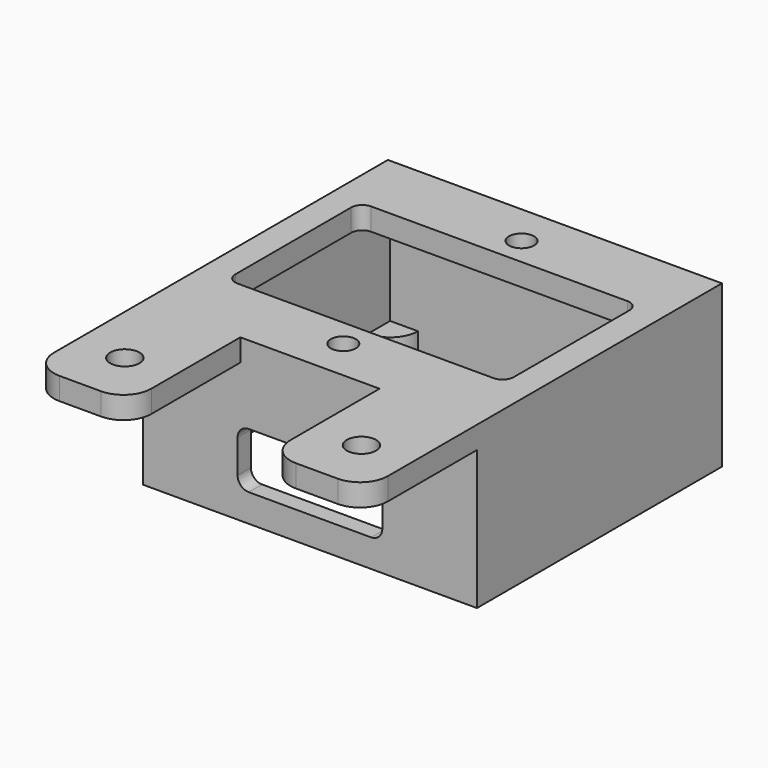
from build123d import *

# Parameters (mm, degrees)
F0_R     = 2.25
F0_R_2   = 2.625
F1_DEPTH = 4
F2_W     = 60
F2_H     = 55
F2_W_2   = 56
F2_H_2   = 50
F3_DEPTH = 25
F5_DEPTH = 25
F6_W     = 5
F6_H     = 5
F7_DEPTH = 5
F8_W     = 56
F8_H     = 50
F9_DEPTH = 2
F10_R    = 4.99999


# Not quite as in the source:
# - a fillet or chamfer is up to 0.001 mm smaller than in the source, because OpenCascade refuses the exact size


with BuildPart() as f1:
    # F0 (on Top) → F1 (new body)
    with BuildSketch(Plane.XY):
        Polygon((30, 27.5), (-30, 27.5), (-30, -27.5), (-12.5000044162, -27.5), (12.5, -27.5), (30, -27.5), align=None)
        with Locations((0, -20)):
            Circle(F0_R, mode=Mode.SUBTRACT)
        with BuildLine():
            ThreePointArc((-25, 13), (-24.4142135624, 14.4142135624), (-23, 15))
            Line((-23, 15), (23, 15))
            ThreePointArc((23, 15), (24.4142135624, 14.4142135624), (25, 13))
            Line((25, 13), (25, -13))
            ThreePointArc((25, -13), (24.4142135624, -14.4142135624), (23, -15))
            Line((23, -15), (-23, -15))
            ThreePointArc((-23, -15), (-24.4142135624, -14.4142135624), (-25, -13))
            Line((-25, -13), (-25, 13))
        make_face(mode=Mode.SUBTRACT)
        with Locations((0, 20)):
            Circle(F0_R, mode=Mode.SUBTRACT)
        with BuildLine():
            Line((-12.5000044162, -27.5), (-30, -27.5))
            Line((-30, -27.5), (-30, -47.5))
            ThreePointArc((-30, -47.5), (-28.5355339059, -51.0355339059), (-25, -52.5))
            Line((-25, -52.5), (-17.5, -52.5))
            ThreePointArc((-17.5, -52.5), (-13.9621173589, -51.0331836094), (-12.5000044162, -47.4933545672))
            Line((-12.5000044162, -47.4933545672), (-12.5000044162, -27.5))
        make_face()
        with Locations((-21.25, -42.5)):
            Circle(F0_R_2, mode=Mode.SUBTRACT)
        with BuildLine():
            Line((30, -47.5), (30, -27.5))
            Line((30, -27.5), (12.5, -27.5))
            Line((12.5, -27.5), (12.5, -47.5))
            ThreePointArc((12.5, -47.5), (13.9644660941, -51.0355339059), (17.5, -52.5))
            Line((17.5, -52.5), (25, -52.5))
            ThreePointArc((25, -52.5), (28.5355339059, -51.0355339059), (30, -47.5))
        make_face()
        with Locations((21.25, -42.5)):
            Circle(F0_R_2, mode=Mode.SUBTRACT)
    extrude(amount=F1_DEPTH)

    # F2 (on face) → F3 (join)
    with BuildSketch(Plane(origin=(0, 0, 0), x_dir=(1, 0, 0), z_dir=(0, 0, -1))):
        Rectangle(F2_W, F2_H)
        with Locations((0, -0.5)):
            Rectangle(F2_W_2, F2_H_2, mode=Mode.SUBTRACT)
    extrude(amount=F3_DEPTH)

    # F4 (on face) → F5 (cut)
    with BuildSketch(Plane(origin=(0, -24.5, 0), x_dir=(-1, 0, 0), z_dir=(0, 1, 0))):
        with BuildLine():
            Line((11, -10), (-11, -10))
            ThreePointArc((-11, -10), (-12.4142135624, -10.5857864376), (-13, -12))
            Line((-13, -12), (-13, -18))
            ThreePointArc((-13, -18), (-12.4142135624, -19.4142135624), (-11, -20))
            Line((-11, -20), (11, -20))
            ThreePointArc((11, -20), (12.4142135624, -19.4142135624), (13, -18))
            Line((13, -18), (13, -12))
            ThreePointArc((13, -12), (12.4142135624, -10.5857864376), (11, -10))
        make_face()
    extrude(amount=-F5_DEPTH, mode=Mode.SUBTRACT)

    # F6 (on face) → F7 (join)
    with BuildSketch(Plane(origin=(0, 0, -25), x_dir=(1, 0, 0), z_dir=(0, 0, -1))):
        with Locations((-25.5, 22)):
            Rectangle(F6_W, F6_H)
        with Locations((25.5, 22)):
            Rectangle(F6_W, F6_H)
        with Locations((25.5, -23)):
            Rectangle(F6_W, F6_H)
        with Locations((-25.5, -23)):
            Rectangle(F6_W, F6_H)
    extrude(amount=-F7_DEPTH)

    # F8 (on face) → F9 (cut)
    with BuildSketch(Plane(origin=(0, 0, -25), x_dir=(1, 0, 0), z_dir=(0, 0, -1))):
        with Locations((0, -0.5)):
            Rectangle(F8_W, F8_H)
    extrude(amount=-F9_DEPTH, mode=Mode.SUBTRACT)

    # F10 (radius 5 in the source; OpenCascade refuses exactly that, so slightly less here)
    f10_edges = [f1.edges().sort_by_distance(p)[0] for p in [
        (-23, -19.5, -21.5),
        (23, -19.5, -21.5),
        (23, 20.5, -21.5),
        (-23, 20.5, -21.5),
    ]]
    fillet(f10_edges, radius=F10_R)


solid = f1.part
